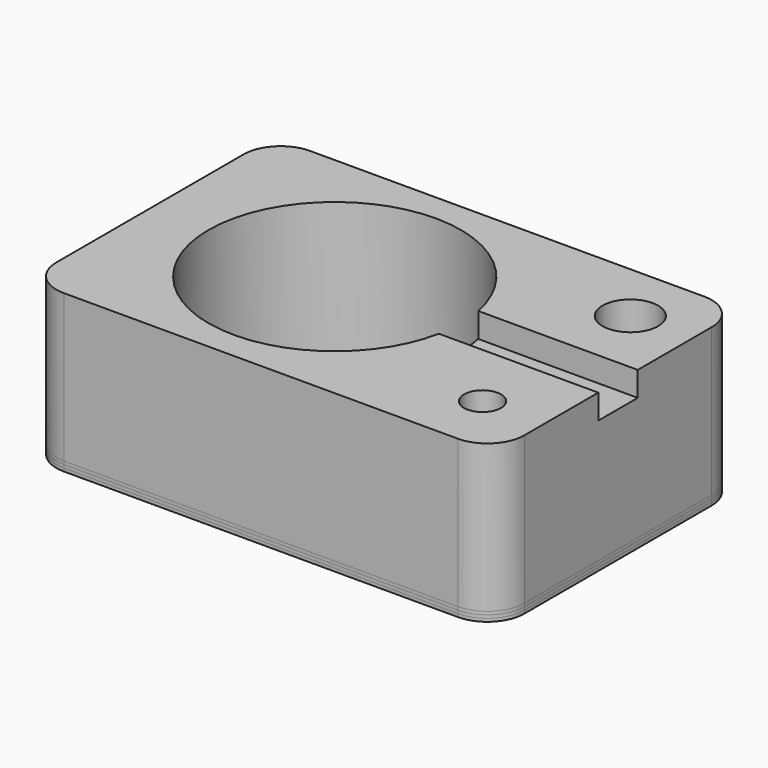
from build123d import *

# Parameters (mm, degrees)
F0_R     = 1.5
F0_R_2   = 10.25
F0_R_3   = 2.2582291175
F1_DEPTH = 12
F3_DEPTH = 2
F4_R     = 2.2582291175
F4_R_2   = 10.25
F4_R_3   = 1.5
F4_R_4   = 5
F5_DEPTH = 0.25
F7_DEPTH = 0.25
F9_DEPTH = 0.25


with BuildPart() as f1:
    # F0 (on Top) → F1 (new body)
    with BuildSketch(Plane.XY):
        with BuildLine():
            Line((-16, -12.5), (16, -12.5))
            ThreePointArc((16, -12.5), (18.1213203436, -11.6213203436), (19, -9.5))
            Line((19, -9.5), (19, 9.5))
            ThreePointArc((19, 9.5), (18.1213203436, 11.6213203436), (16, 12.5))
            Line((16, 12.5), (-16, 12.5))
            ThreePointArc((-16, 12.5), (-18.1213203436, 11.6213203436), (-19, 9.5))
            Line((-19, 9.5), (-19, -9.5))
            ThreePointArc((-19, -9.5), (-18.1213203436, -11.6213203436), (-16, -12.5))
        make_face()
        with Locations((14, -7.5)):
            Circle(F0_R, mode=Mode.SUBTRACT)
        with Locations((-4, 0)):
            Circle(F0_R_2, mode=Mode.SUBTRACT)
        with Locations((14, 7.5)):
            Circle(F0_R_3, mode=Mode.SUBTRACT)
    extrude(amount=F1_DEPTH)

    # F2 (on face) → F3 (cut)
    with BuildSketch(Plane.XY.offset(12)):
        with BuildLine():
            Line((6.0529846314, -2), (19, -2))
            Line((19, -2), (19, 2))
            Line((19, 2), (6.0529846314, 2))
            ThreePointArc((6.0529846314, 2), (6.2006272472, 1.0048401683), (6.25, 0))
            ThreePointArc((6.25, 0), (6.2006272472, -1.0048401683), (6.0529846314, -2))
        make_face()
    extrude(amount=-F3_DEPTH, mode=Mode.SUBTRACT)


with BuildPart() as f5:
    # F4 (on face) → F5 (new body)
    with BuildSketch(Plane(origin=(0, 0, 0), x_dir=(1, 0, 0), z_dir=(0, 0, -1))):
        with BuildLine():
            Line((-16, -12.5), (16, -12.5))
            ThreePointArc((16, -12.5), (18.1213203436, -11.6213203436), (19, -9.5))
            Line((19, -9.5), (19, 9.5))
            ThreePointArc((19, 9.5), (18.1213203436, 11.6213203436), (16, 12.5))
            Line((16, 12.5), (-16, 12.5))
            ThreePointArc((-16, 12.5), (-18.1213203436, 11.6213203436), (-19, 9.5))
            Line((-19, 9.5), (-19, -9.5))
            ThreePointArc((-19, -9.5), (-18.1213203436, -11.6213203436), (-16, -12.5))
        make_face()
        with Locations((14, -7.5)):
            Circle(F4_R, mode=Mode.SUBTRACT)
        with Locations((-4, 0)):
            Circle(F4_R_2, mode=Mode.SUBTRACT)
        with Locations((14, 7.5)):
            Circle(F4_R_3, mode=Mode.SUBTRACT)
        with Locations((-4, 0)):
            Circle(F4_R_2)
        with Locations((-4, 0)):
            Circle(F4_R_4, mode=Mode.SUBTRACT)
        with Locations((14, -7.5)):
            Circle(F4_R)
    extrude(amount=F5_DEPTH)


with BuildPart() as f7:
    # F6 (on face) → F7 (new body)
    with BuildSketch(Plane(origin=(0, 0, -0.25), x_dir=(1, 0, 0), z_dir=(0, 0, -1))):
        with BuildLine():
            Line((-16, -12.5), (16, -12.5))
            ThreePointArc((16, -12.5), (18.1213203436, -11.6213203436), (19, -9.5))
            Line((19, -9.5), (19, 9.5))
            ThreePointArc((19, 9.5), (18.1213203436, 11.6213203436), (16, 12.5))
            Line((16, 12.5), (-16, 12.5))
            ThreePointArc((-16, 12.5), (-18.1213203436, 11.6213203436), (-19, 9.5))
            Line((-19, 9.5), (-19, -9.5))
            ThreePointArc((-19, -9.5), (-18.1213203436, -11.6213203436), (-16, -12.5))
        make_face()
        with BuildLine():
            ThreePointArc((15.5, 7.5), (15.1817562774, 6.5761752867), (14.3620638655, 6.0443524612))
            Line((14.3620638655, 6.0443524612), (4.6269595937, 3.6229356074))
            ThreePointArc((4.6269595937, 3.6229356074), (4.2705878532, 3.2874329762), (4.3713592015, 2.8084674572))
            Line((4.3713592015, 2.8084674572), (6.2525766947, 0.6585046079))
            ThreePointArc((6.2525766947, 0.6585046079), (6.3994234341, -0.4370783525), (5.4472952705, -0.9986101399))
            Line((5.4472952705, -0.9986101399), (0.9417766772, -0.7608175028))
            ThreePointArc((0.9417766772, -0.7608175028), (-9, 0), (0.9417766772, 0.7608175028))
            Line((0.9417766772, 0.7608175028), (2.3648730135, 0.8359258002))
            ThreePointArc((2.3648730135, 0.8359258002), (2.7991253775, 1.1406973672), (2.7148089961, 1.6644831741))
            Line((2.7148089961, 1.6644831741), (1.2474233053, 3.3414953921))
            ThreePointArc((1.2474233053, 3.3414953921), (1.0347168502, 4.261205744), (1.6821849895, 4.9481527404))
            Line((1.6821849895, 4.9481527404), (13.4116409153, 8.8797947628))
            ThreePointArc((13.4116409153, 8.8797947628), (13.5232774843, 8.9222291106), (13.6379361345, 8.9556475388))
            ThreePointArc((13.6379361345, 8.9556475388), (14.9238247133, 8.6817562774), (15.5, 7.5))
        make_face(mode=Mode.SUBTRACT)
        with BuildLine():
            ThreePointArc((0.9417766772, 0.7608175028), (-9, 0), (0.9417766772, -0.7608175028))
            Line((0.9417766772, -0.7608175028), (-3.1610936997, -0.5442758669))
            ThreePointArc((-3.1610936997, -0.5442758669), (-5, 0), (-3.1610936997, 0.5442758669))
            Line((-3.1610936997, 0.5442758669), (0.9417766772, 0.7608175028))
        make_face()
    extrude(amount=F7_DEPTH)


with BuildPart() as f9:
    # F8 (on face) → F9 (new body)
    with BuildSketch(Plane(origin=(0, 0, -0.5), x_dir=(1, 0, 0), z_dir=(0, 0, -1))):
        with BuildLine():
            Line((-16, -12.5), (16, -12.5))
            ThreePointArc((16, -12.5), (18.1213203436, -11.6213203436), (19, -9.5))
            Line((19, -9.5), (19, 9.5))
            ThreePointArc((19, 9.5), (18.1213203436, 11.6213203436), (16, 12.5))
            Line((16, 12.5), (-16, 12.5))
            ThreePointArc((-16, 12.5), (-18.1213203436, 11.6213203436), (-19, 9.5))
            Line((-19, 9.5), (-19, -9.5))
            ThreePointArc((-19, -9.5), (-18.1213203436, -11.6213203436), (-16, -12.5))
        make_face()
        with BuildLine():
            Line((-3.1610936997, 0.5442758669), (2.3648730135, 0.8359258002))
            ThreePointArc((2.3648730135, 0.8359258002), (2.7991253775, 1.1406973672), (2.7148089961, 1.6644831741))
            Line((2.7148089961, 1.6644831741), (1.2474233053, 3.3414953921))
            ThreePointArc((1.2474233053, 3.3414953921), (1.0347168502, 4.261205744), (1.6821849895, 4.9481527404))
            Line((1.6821849895, 4.9481527404), (13.4116409153, 8.8797947628))
            ThreePointArc((13.4116409153, 8.8797947628), (15.4222291106, 7.9767225157), (14.3620638655, 6.0443524612))
            Line((14.3620638655, 6.0443524612), (4.6269595937, 3.6229356074))
            ThreePointArc((4.6269595937, 3.6229356074), (4.2705878532, 3.2874329762), (4.3713592015, 2.8084674572))
            Line((4.3713592015, 2.8084674572), (6.2525766947, 0.6585046079))
            ThreePointArc((6.2525766947, 0.6585046079), (6.3994234341, -0.4370783525), (5.4472952705, -0.9986101399))
            Line((5.4472952705, -0.9986101399), (-3.1610936997, -0.5442758669))
            ThreePointArc((-3.1610936997, -0.5442758669), (-5, 0), (-3.1610936997, 0.5442758669))
        make_face(mode=Mode.SUBTRACT)
        with BuildLine():
            ThreePointArc((2.7148089961, 1.6644831741), (2.7991253775, 1.1406973672), (2.3648730135, 0.8359258002))
            Line((2.3648730135, 0.8359258002), (-3.1610936997, 0.5442758669))
            ThreePointArc((-3.1610936997, 0.5442758669), (-5, 0), (-3.1610936997, -0.5442758669))
            Line((-3.1610936997, -0.5442758669), (5.4472952705, -0.9986101399))
            ThreePointArc((5.4472952705, -0.9986101399), (6.3994234341, -0.4370783525), (6.2525766947, 0.6585046079))
            Line((6.2525766947, 0.6585046079), (4.3713592015, 2.8084674572))
            ThreePointArc((4.3713592015, 2.8084674572), (4.2705878532, 3.2874329762), (4.6269595937, 3.6229356074))
            Line((4.6269595937, 3.6229356074), (14.3620638655, 6.0443524612))
            ThreePointArc((14.3620638655, 6.0443524612), (15.4222291106, 7.9767225157), (13.4116409153, 8.8797947628))
            Line((13.4116409153, 8.8797947628), (1.6821849895, 4.9481527404))
            ThreePointArc((1.6821849895, 4.9481527404), (1.0347168502, 4.261205744), (1.2474233053, 3.3414953921))
            Line((1.2474233053, 3.3414953921), (2.7148089961, 1.6644831741))
        make_face()
    extrude(amount=F9_DEPTH)


solid = Compound([f1.part, f5.part, f7.part, f9.part])
